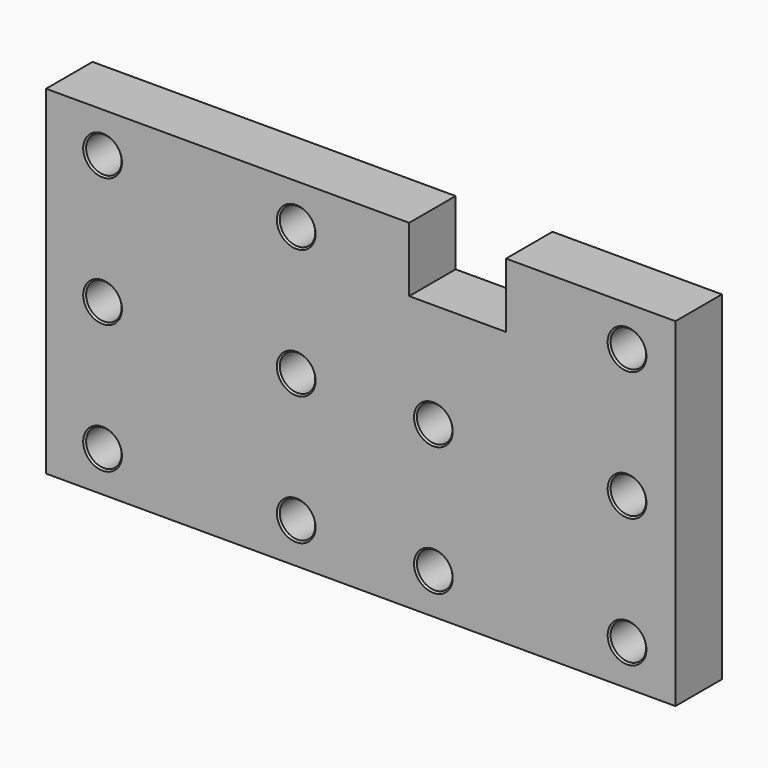
from build123d import *

# Parameters (mm, degrees)
F0_R     = 5.5
F0_W     = 30
F0_H     = 59.6731263399
F0_H_2   = 20
F1_DEPTH = 18
F2_SIZE  = 0.5
F3_W     = 30
F3_H     = 79.6731263399
F4_DEPTH = 25


with BuildPart() as f1:
    # F0 (on Front) → F1 (new body)
    with BuildSketch(Plane.XZ):
        Polygon((-97.5, 52.5), (-97.5, -52.5), (97.5, -52.5), (97.5, 52.5), (45, 52.5), (45, 32.5), (15, 32.5), (15, 52.5), align=None)
        with Locations((-80, -40)):
            Circle(F0_R, mode=Mode.SUBTRACT)
        with Locations((-20, -40)):
            Circle(F0_R, mode=Mode.SUBTRACT)
        with Locations((-80, 0)):
            Circle(F0_R, mode=Mode.SUBTRACT)
        with Locations((-20, 0)):
            Circle(F0_R, mode=Mode.SUBTRACT)
        with Locations((22.5, -40)):
            Circle(F0_R, mode=Mode.SUBTRACT)
        with Locations((82.5, -40)):
            Circle(F0_R, mode=Mode.SUBTRACT)
        with Locations((22.5, 0)):
            Circle(F0_R, mode=Mode.SUBTRACT)
        with Locations((82.5, 0)):
            Circle(F0_R, mode=Mode.SUBTRACT)
        with Locations((-80, 40)):
            Circle(F0_R, mode=Mode.SUBTRACT)
        with Locations((-20, 40)):
            Circle(F0_R, mode=Mode.SUBTRACT)
        with Locations((82.5, 40)):
            Circle(F0_R, mode=Mode.SUBTRACT)
        with Locations((30, 82.33656317)):
            Rectangle(F0_W, F0_H)
        with Locations((30, 42.5)):
            Rectangle(F0_W, F0_H_2)
    extrude(amount=F1_DEPTH)

    # F2
    f2_edges = [f1.edges().sort_by_distance(p)[0] for p in [
        (-74.5, -9, 40),
        (-85.5, 0, 40),
        (-85.5, -18, 40),
        (-74.5, -9, 0),
        (-85.5, 0, 0),
        (-85.5, -18, 0),
        (-74.5, -9, -40),
        (-85.5, 0, -40),
        (-85.5, -18, -40),
        (-14.5, -9, 40),
        (-25.5, 0, 40),
        (-25.5, -18, 40),
        (-14.5, -9, 0),
        (-25.5, 0, 0),
        (-25.5, -18, 0),
        (-14.5, -9, -40),
        (-25.5, 0, -40),
        (-25.5, -18, -40),
        (28, -9, 0),
        (17, 0, 0),
        (17, -18, 0),
        (28, -9, -40),
        (17, 0, -40),
        (17, -18, -40),
        (88, -9, 40),
        (77, 0, 40),
        (77, -18, 40),
        (88, -9, 0),
        (77, 0, 0),
        (77, -18, 0),
        (88, -9, -40),
        (77, 0, -40),
        (77, -18, -40),
    ]]
    chamfer(f2_edges, length=F2_SIZE)

    # F3 (on face) → F4 (cut)
    with BuildSketch(Plane.XZ.offset(18)):
        with Locations((30, 72.33656317)):
            Rectangle(F3_W, F3_H)
    extrude(amount=-F4_DEPTH, mode=Mode.SUBTRACT)


solid = f1.part
